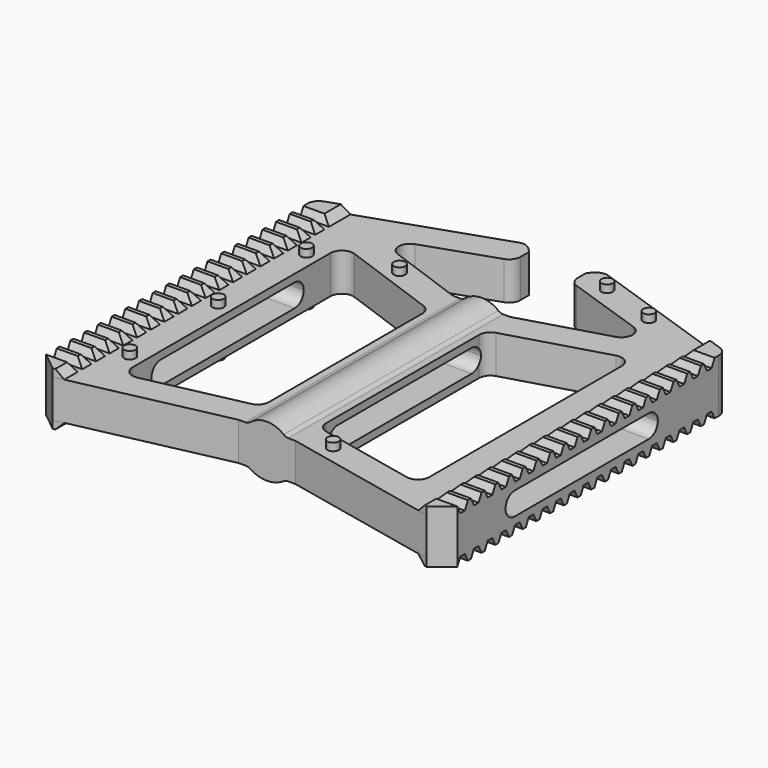
from build123d import *

# Parameters (mm, degrees)
F1_DEPTH       = 10
F3_DEPTH       = 25
F4_SIZE        = 5
F5_R           = 3
F7_DEPTH       = 2
F7_DEPTH_BACK  = 12
F8_DEPTH       = 2
F10_DEPTH      = 2
F10_DEPTH_BACK = 12
F11_SIZE       = 1.99999
F12_R          = 1.5
F13_DEPTH      = 2
F13_DEPTH_BACK = 12
F15_DEPTH      = 70.5
F16_R          = 2
F19_DEPTH      = 54.001
F19_DEPTH_BACK = 54.001
F21_DEPTH      = 8
F23_DEPTH      = 8


# Not quite as in the source:
# - a fillet or chamfer is up to 0.001 mm smaller than in the source, because OpenCascade refuses the exact size


with BuildPart() as f1:
    # F0 (on Top) → F1 (new body)
    with BuildSketch(Plane.XY):
        Polygon((64, 108), (44, 108), (0, 93), (0, 0), (46.5, 10), (61.5, 10), (108, 0), (108, 93), align=None)
    extrude(amount=F1_DEPTH)

    # F2 (on face) → F3 (cut)
    with BuildSketch(Plane.XY.offset(10)):
        Polygon((46.5, 72.5266522312), (15, 83.8932790255), (15, 10.897276768), (46.5, 17.6714703164), align=None)
        Polygon((93, 81.7880158676), (61.5, 72.5266522312), (61.5, 17.6714703164), (93, 10.897276768), align=None)
        Polygon((46.5, 100.5), (18, 90.7840909091), (46.5, 80.5), (61.5, 80.5), (93, 89.7613636364), (61.5, 100.5), (61.5, 105.5), (64, 108), (44, 108), (46.5, 105.5), align=None)
    extrude(amount=-F3_DEPTH, mode=Mode.SUBTRACT)

    # F4
    f4_edges = [f1.edges().sort_by_distance(p)[0] for p in [
        (0, 0, 5),
        (108, 0, 5),
    ]]
    chamfer(f4_edges, length=F4_SIZE)

    # F5
    f5_edges = [f1.edges().sort_by_distance(p)[0] for p in [
        (46.5, 17.67147, 5),
        (93, 10.897277, 5),
        (46.5, 80.5, 5),
        (61.5, 80.5, 5),
        (61.5, 17.67147, 5),
        (15, 10.897277, 5),
        (93, 81.788016, 5),
        (46.5, 72.526652, 5),
        (15, 83.893279, 5),
        (93, 89.761364, 5),
        (18, 90.784091, 5),
        (61.5, 72.526652, 5),
        (108, 93, 5),
        (0, 93, 5),
        (64, 108, 5),
        (44, 108, 5),
        (61.5, 100.5, 5),
        (46.5, 100.5, 5),
    ]]
    fillet(f5_edges, radius=F5_R)

    # F6 (on face) → F7 (join, two sides)
    with BuildSketch(Plane.XY.offset(10)) as f7_sk:
        with BuildLine():
            Line((105.9680217834, 93.6927198466), (100.5, 95.5568181818))
            Line((100.5, 95.5568181818), (100.5, 1.6129032258))
            Line((100.5, 1.6129032258), (103.1117584435, 1.0512347433))
            Line((103.1117584435, 1.0512347433), (108, 5))
            Line((108, 5), (108, 90.853189282))
            ThreePointArc((108, 90.853189282), (107.4396788057, 92.5990321515), (105.9680217834, 93.6927198466))
        make_face()
    extrude(amount=F7_DEPTH)
    extrude(f7_sk.sketch, amount=-F7_DEPTH_BACK)

    # F6 (on face) → F8 (join)
    with BuildSketch(Plane.XY.offset(10)):
        with BuildLine():
            Line((105.9680217834, 93.6927198466), (100.5, 95.5568181818))
            Line((100.5, 95.5568181818), (100.5, 1.6129032258))
            Line((100.5, 1.6129032258), (103.1117584435, 1.0512347433))
            Line((103.1117584435, 1.0512347433), (108, 5))
            Line((108, 5), (108, 90.853189282))
            ThreePointArc((108, 90.853189282), (107.4396788057, 92.5990321515), (105.9680217834, 93.6927198466))
        make_face()
    extrude(amount=F8_DEPTH)

    # F9 (on face) → F10 (join, two sides)
    with BuildSketch(Plane(origin=(0, 0, 0), x_dir=(1, 0, 0), z_dir=(0, 0, -1))) as f10_sk:
        with BuildLine():
            Line((2.0319782166, -93.6927198466), (7.5, -95.5568181818))
            Line((7.5, -95.5568181818), (7.5, -1.6129032258))
            Line((7.5, -1.6129032258), (4.8882415565, -1.0512347433))
            Line((4.8882415565, -1.0512347433), (0, -5))
            Line((0, -5), (0, -90.853189282))
            ThreePointArc((0, -90.853189282), (0.5603211943, -92.5990321515), (2.0319782166, -93.6927198466))
        make_face()
    extrude(amount=F10_DEPTH)
    extrude(f10_sk.sketch, amount=-F10_DEPTH_BACK)

    # F11 (size 2 in the source; OpenCascade refuses exactly that, so slightly less here)
    f11_edges = [f1.edges().sort_by_distance(p)[0] for p in [
        (100.5, 48.584861, 12),
        (7.5, 48.584861, -2),
        (100.5, 48.584861, -2),
        (7.5, 48.584861, 12),
    ]]
    chamfer(f11_edges, length=F11_SIZE)

    # F12 (on face) → F13 (join, two sides)
    with BuildSketch(Plane.XY.offset(10)) as f13_sk:
        with Locations((69.5, 102.3358173321)):
            Circle(F12_R)
        with Locations((84.5, 97.3135693139)):
            Circle(F12_R)
        with Locations((69.5, 12.3710207279)):
            Circle(F12_R)
        with Locations((11.5, 76.1214040328)):
            Circle(F12_R)
        with Locations((11.5, 47.1214040328)):
            Circle(F12_R)
        with Locations((11.5, 18.1110261849)):
            Circle(F12_R)
        with Locations((31.5, 81.6602272825)):
            Circle(F12_R)
    extrude(amount=F13_DEPTH)
    extrude(f13_sk.sketch, amount=-F13_DEPTH_BACK)

    # F14 (on face) → F15 (join, through all)
    with BuildSketch(Plane.XZ.offset(-10)):
        with BuildLine():
            Line((49.1010205144, 10), (58.8989794856, 10))
            ThreePointArc((58.8989794856, 10), (54, 12), (49.1010205144, 10))
        make_face()
        with BuildLine():
            ThreePointArc((49.1010205144, 0), (54, -1.6754446797), (58.8989794856, 0))
            Line((58.8989794856, 0), (49.1010205144, 0))
        make_face()
    extrude(amount=-F15_DEPTH)

    # F16
    f16_edges = [f1.edges().sort_by_distance(p)[0] for p in [
        (49.101021, 45.25, 0),
        (58.898979, 45.25, 10),
        (58.898979, 45.25, 0),
        (49.101021, 45.25, 10),
    ]]
    fillet(f16_edges, radius=F16_R)

    # F18 (on offset) → F19 (cut, two sides)
    with BuildSketch(Plane(origin=(54, 0, 0), x_dir=(0, -1, 0), z_dir=(-1, 0, 0))) as f19_sk:
        with BuildLine():
            Line((-23.853189282, 8), (-67.853189282, 8))
            ThreePointArc((-67.853189282, 8), (-69.9745096256, 7.1213203436), (-70.853189282, 5))
            ThreePointArc((-70.853189282, 5), (-69.9745096256, 2.8786796564), (-67.853189282, 2))
            Line((-67.853189282, 2), (-23.853189282, 2))
            ThreePointArc((-23.853189282, 2), (-21.7318689385, 2.8786796564), (-20.853189282, 5))
            ThreePointArc((-20.853189282, 5), (-21.7318689385, 7.1213203436), (-23.853189282, 8))
        make_face()
    extrude(amount=-F19_DEPTH, mode=Mode.SUBTRACT)
    extrude(f19_sk.sketch, amount=F19_DEPTH_BACK, mode=Mode.SUBTRACT)

    # F20 (on face) → F21 (cut)
    with BuildSketch(Plane(origin=(0, 0, 0), x_dir=(0, -1, 0), z_dir=(-1, 0, 0))):
        Polygon((-87, 10), (-86, 12), (-89.5, 12), (-88.5, 10), align=None)
        Polygon((-82.5, 10), (-81.5, 12), (-85, 12), (-84, 10), align=None)
        Polygon((-78, 10), (-77, 12), (-80.5, 12), (-79.5, 10), align=None)
        Polygon((-73.5, 10), (-72.5, 12), (-76, 12), (-75, 10), align=None)
        Polygon((-69, 10), (-68, 12), (-71.5, 12), (-70.5, 10), align=None)
        Polygon((-64.5, 10), (-63.5, 12), (-67, 12), (-66, 10), align=None)
        Polygon((-60, 10), (-59, 12), (-62.5, 12), (-61.5, 10), align=None)
        Polygon((-55.5, 10), (-54.5, 12), (-58, 12), (-57, 10), align=None)
        Polygon((-51, 10), (-50, 12), (-53.5, 12), (-52.5, 10), align=None)
        Polygon((-46.5, 10), (-45.5, 12), (-49, 12), (-48, 10), align=None)
        Polygon((-42, 10), (-41, 12), (-44.5, 12), (-43.5, 10), align=None)
        Polygon((-37.5, 10), (-36.5, 12), (-40, 12), (-39, 10), align=None)
        Polygon((-33, 10), (-32, 12), (-35.5, 12), (-34.5, 10), align=None)
        Polygon((-28.5, 10), (-27.5, 12), (-31, 12), (-30, 10), align=None)
        Polygon((-24, 10), (-23, 12), (-26.5, 12), (-25.5, 10), align=None)
        Polygon((-19.5, 10), (-18.5, 12), (-22, 12), (-21, 10), align=None)
        Polygon((-15, 10), (-14, 12), (-17.5, 12), (-16.5, 10), align=None)
        Polygon((-10.5, 10), (-9.5, 12), (-13, 12), (-12, 10), align=None)
        Polygon((-6, 10), (-5, 12), (-8.5, 12), (-7.5, 10), align=None)
        Polygon((-89.5, -2), (-86, -2), (-87, 0), (-88.5, 0), align=None)
        Polygon((-85, -2), (-81.5, -2), (-82.5, 0), (-84, 0), align=None)
        Polygon((-80.5, -2), (-77, -2), (-78, 0), (-79.5, 0), align=None)
        Polygon((-76, -2), (-72.5, -2), (-73.5, 0), (-75, 0), align=None)
        Polygon((-71.5, -2), (-68, -2), (-69, 0), (-70.5, 0), align=None)
        Polygon((-67, -2), (-63.5, -2), (-64.5, 0), (-66, 0), align=None)
        Polygon((-62.5, -2), (-59, -2), (-60, 0), (-61.5, 0), align=None)
        Polygon((-58, -2), (-54.5, -2), (-55.5, 0), (-57, 0), align=None)
        Polygon((-53.5, -2), (-50, -2), (-51, 0), (-52.5, 0), align=None)
        Polygon((-49, -2), (-45.5, -2), (-46.5, 0), (-48, 0), align=None)
        Polygon((-44.5, -2), (-41, -2), (-42, 0), (-43.5, 0), align=None)
        Polygon((-40, -2), (-36.5, -2), (-37.5, 0), (-39, 0), align=None)
        Polygon((-35.5, -2), (-32, -2), (-33, 0), (-34.5, 0), align=None)
        Polygon((-31, -2), (-27.5, -2), (-28.5, 0), (-30, 0), align=None)
        Polygon((-26.5, -2), (-23, -2), (-24, 0), (-25.5, 0), align=None)
        Polygon((-22, -2), (-18.5, -2), (-19.5, 0), (-21, 0), align=None)
        Polygon((-17.5, -2), (-14, -2), (-15, 0), (-16.5, 0), align=None)
        Polygon((-13, -2), (-9.5, -2), (-10.5, 0), (-12, 0), align=None)
        Polygon((-8.5, -2), (-5, -2), (-6, 0), (-7.5, 0), align=None)
    extrude(amount=-F21_DEPTH, mode=Mode.SUBTRACT)

    # F22 (on face) → F23 (cut)
    with BuildSketch(Plane.YZ.offset(108)):
        Polygon((8.5, 12), (5, 12), (6, 10), (7.5, 10), align=None)
        Polygon((13, 12), (9.5, 12), (10.5, 10), (12, 10), align=None)
        Polygon((17.5, 12), (14, 12), (15, 10), (16.5, 10), align=None)
        Polygon((22, 12), (18.5, 12), (19.5, 10), (21, 10), align=None)
        Polygon((26.5, 12), (23, 12), (24, 10), (25.5, 10), align=None)
        Polygon((31, 12), (27.5, 12), (28.5, 10), (30, 10), align=None)
        Polygon((35.5, 12), (32, 12), (33, 10), (34.5, 10), align=None)
        Polygon((40, 12), (36.5, 12), (37.5, 10), (39, 10), align=None)
        Polygon((44.5, 12), (41, 12), (42, 10), (43.5, 10), align=None)
        Polygon((49, 12), (45.5, 12), (46.5, 10), (48, 10), align=None)
        Polygon((53.5, 12), (50, 12), (51, 10), (52.5, 10), align=None)
        Polygon((58, 12), (54.5, 12), (55.5, 10), (57, 10), align=None)
        Polygon((62.5, 12), (59, 12), (60, 10), (61.5, 10), align=None)
        Polygon((67, 12), (63.5, 12), (64.5, 10), (66, 10), align=None)
        Polygon((71.5, 12), (68, 12), (69, 10), (70.5, 10), align=None)
        Polygon((76, 12), (72.5, 12), (73.5, 10), (75, 10), align=None)
        Polygon((80.5, 12), (77, 12), (78, 10), (79.5, 10), align=None)
        Polygon((85, 12), (81.5, 12), (82.5, 10), (84, 10), align=None)
        Polygon((89.5, 12), (86, 12), (87, 10), (88.5, 10), align=None)
        Polygon((12, 0), (10.5, 0), (9.5, -2), (13, -2), align=None)
        Polygon((7.5, 0), (6, 0), (5, -2), (8.5, -2), align=None)
        Polygon((26.5, -2), (25.5, 0), (24, 0), (23, -2), align=None)
        Polygon((87, 0), (86, -2), (89.5, -2), (88.5, 0), align=None)
        Polygon((33, 0), (32, -2), (35.5, -2), (34.5, 0), align=None)
        Polygon((51, 0), (50, -2), (53.5, -2), (52.5, 0), align=None)
        Polygon((69, 0), (68, -2), (71.5, -2), (70.5, 0), align=None)
        Polygon((42, 0), (41, -2), (44.5, -2), (43.5, 0), align=None)
        Polygon((60, 0), (59, -2), (62.5, -2), (61.5, 0), align=None)
        Polygon((78, 0), (77, -2), (80.5, -2), (79.5, 0), align=None)
        Polygon((84, 0), (82.5, 0), (81.5, -2), (85, -2), align=None)
        Polygon((30, 0), (28.5, 0), (27.5, -2), (31, -2), align=None)
        Polygon((48, 0), (46.5, 0), (45.5, -2), (49, -2), align=None)
        Polygon((66, 0), (64.5, 0), (63.5, -2), (67, -2), align=None)
        Polygon((39, 0), (37.5, 0), (36.5, -2), (40, -2), align=None)
        Polygon((57, 0), (55.5, 0), (54.5, -2), (58, -2), align=None)
        Polygon((75, 0), (73.5, 0), (72.5, -2), (76, -2), align=None)
        Polygon((19.5, 0), (18.5, -2), (22, -2), (21, 0), align=None)
        Polygon((16.5, 0), (15, 0), (14, -2), (17.5, -2), align=None)
    extrude(amount=-F23_DEPTH, mode=Mode.SUBTRACT)


solid = f1.part
